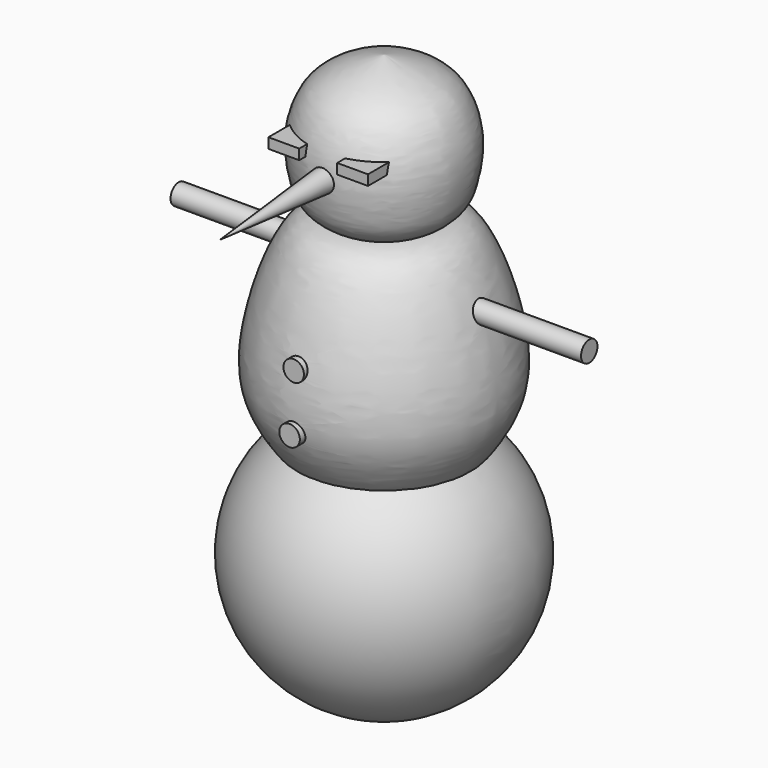
from build123d import *

# Parameters (mm, degrees)
F6_W      = 3.81
F6_H      = 1.27
F7_DEPTH  = 10.16
F8_W      = 3.81
F8_H      = 1.27
F9_DEPTH  = 10.16
F10_R     = 2.2225
F12_R     = 1.27
F13_DEPTH = 25.4
F14_R     = 1.27
F15_DEPTH = 25.4
F16_R     = 1.27
F17_DEPTH = 13.97
F18_R     = 1.27
F19_DEPTH = 14.605


# Not quite as in the source:
# - an extrude whose draft closes it to a point is written as a loft to that point
# - a feature names something its author has since deleted; it is built from what else it names


with BuildPart() as f1:
    # F0 (on Front) → F1 (revolve)
    with BuildSketch(Plane.XZ):
        with BuildLine():
            add(Edge.make_bspline(
                [(0, 2.8886205982), (6.6735734029, 2.641451239), (10.3540448543, 2.3475350303), (15.1586673121, -13.1854203701), (12.4171703884, -20.9762656209), (7.2802522915, -26.8015097962), (0, -27.0711500198)],
                knots=[0, 0, 0, 0, 0.2413494897, 0.514493962, 0.7235907814, 1, 1, 1, 1], degree=3))
            Line((0, 2.8886205982), (0, -27.0711500198))
        make_face()
    revolve(axis=Axis((0, 0, 2.1519046277), (0, 0, -1)))

    # F12 (on Right) → F13 (join)
    with BuildSketch(Plane.YZ):
        with Locations((0, -4.4712037779)):
            Circle(F12_R)
    extrude(amount=F13_DEPTH)

    # F14 (on Right) → F15 (join)
    with BuildSketch(Plane.YZ):
        with Locations((0, -3.8473161403)):
            Circle(F14_R)
    extrude(amount=-F15_DEPTH)

    # F16 (on Front) → F17 (join)
    with BuildSketch(Plane.XZ):
        with Locations((0, -9.1882972047)):
            Circle(F16_R)
    extrude(amount=F17_DEPTH)

    # F18 (on Front) → F19 (join)
    with BuildSketch(Plane.XZ):
        with Locations((0, -15.9874036908)):
            Circle(F18_R)
    extrude(amount=F19_DEPTH)


with BuildPart() as f3:
    # F2 (on Front) → F3 (revolve)
    with BuildSketch(Plane.XZ):
        with BuildLine():
            add(Edge.make_bspline(
                [(0, 19.5875093341), (6.1392970383, 18.1140769273), (8.6585873557, 15.251758349), (9.8517482862, 10.5322369407), (9.1128004555, 5.0161565335), (7.6127294451, 2.1519048605), (0, 0)],
                knots=[0, 0, 0, 0, 0.2988485598, 0.488814017, 0.6878817535, 1, 1, 1, 1], degree=3))
            Line((0, 19.5875093341), (0, 0))
        make_face()
    revolve(axis=Axis((0, 0, 0.1873299479), (0, 0, -1)))

    # F6 (on Front) → F7 (join)
    with BuildSketch(Plane.XZ):
        with Locations((-4.26982732, 12.0650008863)):
            Rectangle(F6_W, F6_H)
    extrude(amount=F7_DEPTH)

    # F8 (on Front) → F9 (join)
    with BuildSketch(Plane.XZ):
        with Locations((4.2420482496, 12.03115104)):
            Rectangle(F8_W, F8_H)
    extrude(amount=F9_DEPTH)


with BuildPart() as f5:
    # F4 (on Front) → F5 (revolve)
    with BuildSketch(Plane.XZ):
        with BuildLine():
            ThreePointArc((0, -51.0408654809), (16.356726177, -34.6841393039), (0, -18.3274131268))
            Line((0, -18.3274131268), (0, -51.0408654809))
        make_face()
    revolve(axis=Axis((0, 0, -16.2659883499), (0, 0, -1)))


with BuildPart() as f11:
    # F10 (on Front) → F11 section 0
    with BuildSketch(Plane.XZ, mode=Mode.PRIVATE) as f11_s0:
        with Locations((0, 9.7145279869)):
            Circle(F10_R)
    loft([f11_s0.sketch, Vertex(0, -25.4032912429, 9.7145279869)], ruled=True)


solid = Compound([f1.part, f3.part, f5.part, f11.part])
